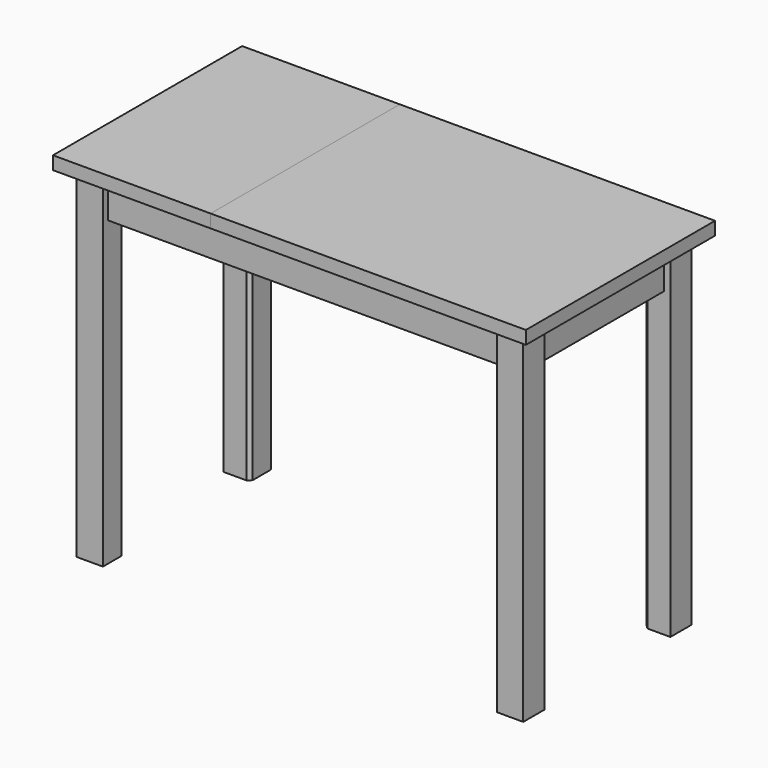
from build123d import *

# Parameters (mm, degrees)
F0_W     = 609.6
F0_H     = 457.2
F1_DEPTH = 25.4
F0_W_2   = 304.8
F2_DEPTH = 25.4
F3_W     = 6.7882202148
F3_H     = 355.6
F3_W_2   = 5.9117797852
F4_DEPTH = 76.2
F5_DEPTH = 660.4


with BuildPart() as f1:
    # F0 (on Top) → F1 (new body)
    with BuildSketch(Plane.XY):
        with Locations((-89.3258527756, 10.1408557653)):
            Rectangle(F0_W, F0_H)
    extrude(amount=F1_DEPTH)


with BuildPart() as f2:
    # F0 (on Top) → F2 (new body)
    with BuildSketch(Plane.XY):
        with Locations((-546.5258527756, 10.1408557653)):
            Rectangle(F0_W_2, F0_H)
    extrude(amount=F2_DEPTH)


with BuildPart() as f4:
    # F3 (on face) → F4 (new body)
    with BuildSketch(Plane.XY):
        Polygon((-394.1258527756, -167.6591442347), (-394.1258527756, -180.3591442347), (139.2741472244, -180.3591442347), (139.2741472244, -167.6591442347), (120.2241472244, -167.6591442347), (102.2636349823, -167.6591442347), (-241.7258527756, -167.6591442347), (-388.2140729904, -167.6591442347), align=None)
        Polygon((-622.7258527756, -167.6591442347), (-622.7258527756, -180.3591442347), (-394.1258527756, -180.3591442347), (-394.1258527756, -167.6591442347), (-400.9140729904, -167.6591442347), (-585.7153405334, -167.6591442347), (-603.6758527756, -167.6591442347), align=None)
        Polygon((-622.7258527756, -142.2591442347), (-622.7258527756, -148.6091442347), (-603.6758527756, -167.6591442347), (-585.7153405334, -167.6591442347), (-648.1258527756, -105.2486319925), (-648.1258527756, -123.2091442347), (-629.0758527756, -142.2591442347), align=None)
        Polygon((-660.8258527756, 162.5408557653), (-660.8258527756, -142.2591442347), (-648.1258527756, -142.2591442347), (-648.1258527756, -123.2091442347), (-648.1258527756, -105.2486319925), (-648.1258527756, 125.5303435232), (-648.1258527756, 143.4908557653), (-648.1258527756, 162.5408557653), align=None)
        Polygon((-622.7258527756, 162.5408557653), (-629.0758527756, 162.5408557653), (-648.1258527756, 143.4908557653), (-648.1258527756, 125.5303435232), (-585.7153405334, 187.9408557653), (-603.6758527756, 187.9408557653), (-622.7258527756, 168.8908557653), align=None)
        Polygon((-400.9140729904, 187.9408557653), (-394.1258527756, 187.9408557653), (-394.1258527756, 200.6408557653), (-622.7258527756, 200.6408557653), (-622.7258527756, 187.9408557653), (-603.6758527756, 187.9408557653), (-585.7153405334, 187.9408557653), align=None)
        Polygon((-394.1258527756, 200.6408557653), (-394.1258527756, 187.9408557653), (-388.2140729904, 187.9408557653), (102.2636349823, 187.9408557653), (120.2241472244, 187.9408557653), (139.2741472244, 187.9408557653), (139.2741472244, 200.6408557653), align=None)
        Polygon((120.2241472244, 187.9408557653), (102.2636349823, 187.9408557653), (164.6741472244, 125.5303435232), (164.6741472244, 143.4908557653), (145.6241472244, 162.5408557653), (139.2741472244, 162.5408557653), (139.2741472244, 168.8908557653), align=None)
        Polygon((164.6741472244, -142.2591442347), (177.3741472244, -142.2591442347), (177.3741472244, 162.5408557653), (164.6741472244, 162.5408557653), (164.6741472244, 143.4908557653), (164.6741472244, 125.5303435232), (164.6741472244, -105.2486319925), (164.6741472244, -123.2091442347), align=None)
        Polygon((-629.0758527756, -142.2591442347), (-622.7258527756, -148.6091442347), (-622.7258527756, -142.2591442347), align=None)
        Polygon((-622.7258527756, 168.8908557653), (-629.0758527756, 162.5408557653), (-622.7258527756, 162.5408557653), align=None)
        Polygon((145.6241472244, 162.5408557653), (139.2741472244, 168.8908557653), (139.2741472244, 162.5408557653), align=None)
        Polygon((139.2741472244, -142.2591442347), (139.2741472244, -148.6091442347), (145.6241472244, -142.2591442347), align=None)
        Polygon((120.2241472244, -167.6591442347), (139.2741472244, -148.6091442347), (139.2741472244, -142.2591442347), (145.6241472244, -142.2591442347), (164.6741472244, -123.2091442347), (164.6741472244, -105.2486319925), (102.2636349823, -167.6591442347), align=None)
        with Locations((-397.519962883, 10.1408557653)):
            Rectangle(F3_W, F3_H)
        with Locations((-391.169962883, 10.1408557653)):
            Rectangle(F3_W_2, F3_H)
    extrude(amount=-F4_DEPTH)

    # F3 (on face) → F5 (join)
    with BuildSketch(Plane.XY):
        Polygon((139.2741472244, 213.3408557653), (139.2741472244, 200.6408557653), (139.2741472244, 187.9408557653), (139.2741472244, 168.8908557653), (145.6241472244, 162.5408557653), (164.6741472244, 162.5408557653), (177.3741472244, 162.5408557653), (190.0741472244, 162.5408557653), (190.0741472244, 213.3408557653), align=None)
        Polygon((139.2741472244, -167.6591442347), (139.2741472244, -180.3591442347), (139.2741472244, -193.0591442347), (190.0741472244, -193.0591442347), (190.0741472244, -142.2591442347), (177.3741472244, -142.2591442347), (164.6741472244, -142.2591442347), (145.6241472244, -142.2591442347), (139.2741472244, -148.6091442347), align=None)
        Polygon((-673.5258527756, 162.5408557653), (-660.8258527756, 162.5408557653), (-648.1258527756, 162.5408557653), (-629.0758527756, 162.5408557653), (-622.7258527756, 168.8908557653), (-622.7258527756, 187.9408557653), (-622.7258527756, 200.6408557653), (-622.7258527756, 213.3408557653), (-673.5258527756, 213.3408557653), align=None)
        Polygon((-673.5258527756, -142.2591442347), (-673.5258527756, -193.0591442347), (-622.7258527756, -193.0591442347), (-622.7258527756, -180.3591442347), (-622.7258527756, -167.6591442347), (-622.7258527756, -148.6091442347), (-629.0758527756, -142.2591442347), (-648.1258527756, -142.2591442347), (-660.8258527756, -142.2591442347), align=None)
    extrude(amount=-F5_DEPTH)


solid = Compound([f1.part, f2.part, f4.part])
